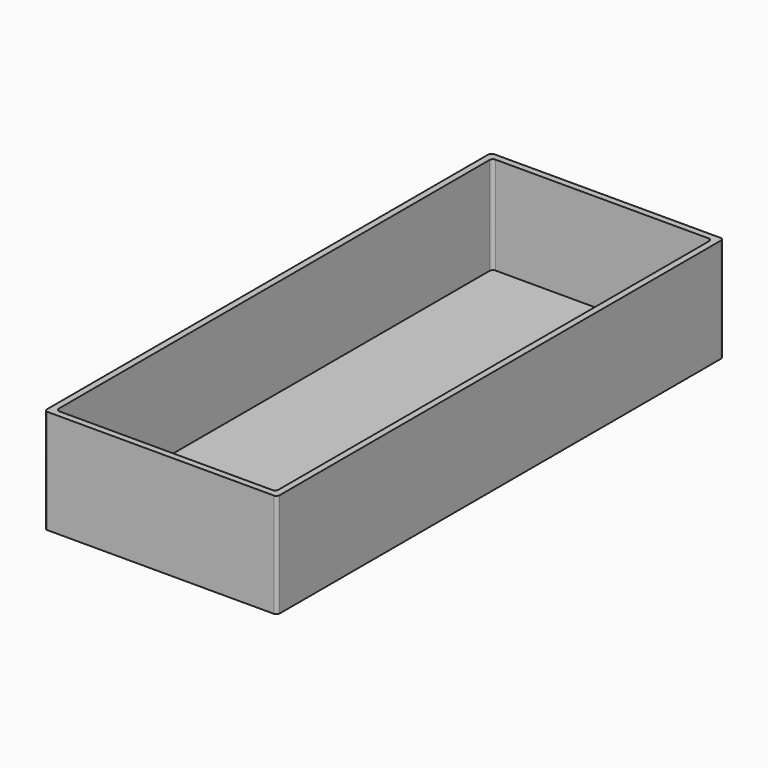
from build123d import *

# Parameters (mm, degrees)
F2_DEPTH = 40.64
F4_DEPTH = 38.1


# Not quite as in the source:
# - a variable given as a bare number and used for a length is read in inches; the dataset says mm whatever the document's units were


with BuildPart() as f2:
    # F1 (on Top) → F2 (new body)
    with BuildSketch(Plane.XY):
        with BuildLine():
            ThreePointArc((0, 1.27), (0.3719743879, 0.3719743879), (1.27, 0))
            Line((1.27, 0), (89.535, 0))
            ThreePointArc((89.535, 0), (90.4330256121, 0.3719743879), (90.805, 1.27))
            Line((90.805, 1.27), (90.805, 216.535))
            ThreePointArc((90.805, 216.535), (90.4330256121, 217.4330256121), (89.535, 217.805))
            Line((89.535, 217.805), (1.27, 217.805))
            ThreePointArc((1.27, 217.805), (0.3719743879, 217.4330256121), (0, 216.535))
            Line((0, 216.535), (0, 1.27))
        make_face()
    extrude(amount=F2_DEPTH)

    # F3 (on face) → F4 (cut)
    with BuildSketch(Plane.XY.offset(40.64)):
        with BuildLine():
            Line((2.54, 213.995), (2.54, 3.81))
            ThreePointArc((2.54, 3.81), (2.9119743879, 2.9119743879), (3.81, 2.54))
            Line((3.81, 2.54), (86.995, 2.54))
            ThreePointArc((86.995, 2.54), (87.8930256121, 2.9119743879), (88.265, 3.81))
            Line((88.265, 3.81), (88.265, 213.995))
            ThreePointArc((88.265, 213.995), (87.8930256121, 214.8930256121), (86.995, 215.265))
            Line((86.995, 215.265), (3.81, 215.265))
            ThreePointArc((3.81, 215.265), (2.9119743879, 214.8930256121), (2.54, 213.995))
        make_face()
    extrude(amount=-F4_DEPTH, mode=Mode.SUBTRACT)


solid = f2.part
